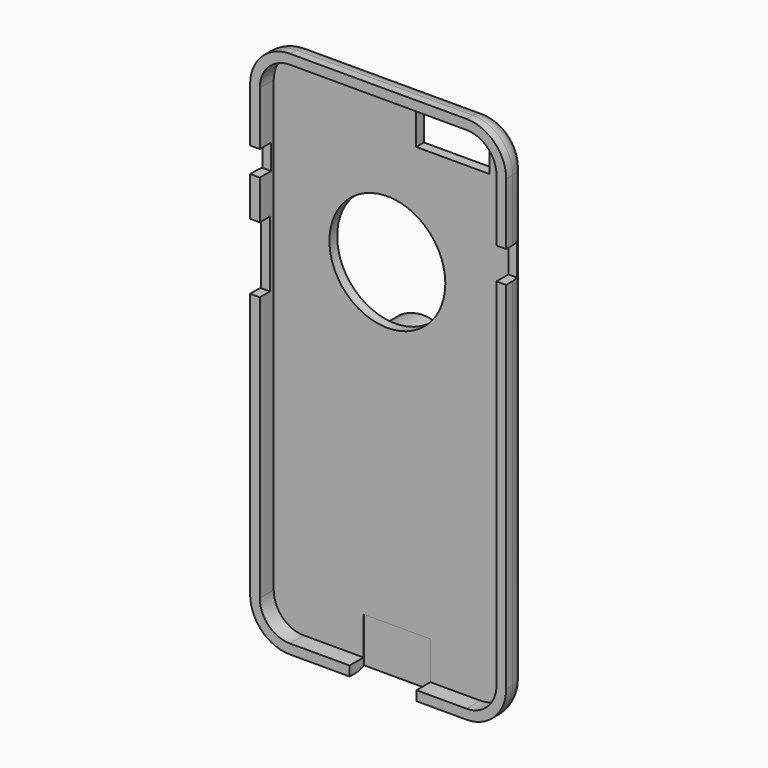
from build123d import *

# Parameters (mm, degrees)
F0_W          = 67.1
F0_H          = 138.6
F1_DEPTH      = 7.1
F2_R          = 10.4245741623
F3_T          = -2.54
F4_W          = 19.2213095725
F4_H          = 9.1803260148
F5_DEPTH      = 12.5
F6_W          = 17.5000010058
F6_H          = 4.661475262
F7_DEPTH      = 12.5
F8_W          = 3.0759498477
F8_H          = 14.1388773918
F9_DEPTH      = 12.5
F10_W         = 3.7169439722
F10_H         = 6.5781623125
F11_DEPTH     = 12.5
F12_W         = 3.3410489097
F12_H         = 17.2911705449
F13_DEPTH     = 12.5
F14_W         = 3.904892784
F14_H         = 8.2696899772
F15_DEPTH     = 12.5
F16_T1_DEPTH  = 117.7508516753
F16_T3_DEPTH  = 46.2508516753
F16_T6_ANGLE  = 90
F16_T8_ANGLE  = 90
F16_T10_ANGLE = 90
F16_T12_ANGLE = 90
F17_R         = 15.1895589548
F18_DEPTH     = 12.5
F19_R         = 10.4830955048
F19_R_2       = 9.0277735867
F20_DEPTH     = 7.7


# Not quite as in the source:
# - a fillet or chamfer that OpenCascade refuses, or shapes differently, is made with other operations: its cross-section is extruded or revolved along the edge and cut away or added


with BuildPart() as f1:
    # F0 (on Front) → F1 (new body)
    with BuildSketch(Plane.XZ):
        Rectangle(F0_W, F0_H)
    extrude(amount=F1_DEPTH)

    # F2
    f2_edges = [f1.edges().sort_by_distance(p)[0] for p in [
        (33.55, -3.55, 69.3),
        (-33.55, -3.55, 69.3),
        (-33.55, -3.55, -69.3),
        (33.55, -3.55, -69.3),
    ]]
    fillet(f2_edges, radius=F2_R)

    # F3
    f3_openings = [f1.faces().sort_by_distance(p)[0] for p in [
        (0, -7.1, 0),
    ]]
    offset(amount=F3_T, openings=f3_openings)

    # F4 (on Front) → F5 (cut, symmetric)
    with BuildSketch(Plane.XZ):
        with Locations((15.9221310169, 60.1024609059)):
            Rectangle(F4_W, F4_H)
    extrude(amount=F5_DEPTH, both=True, mode=Mode.SUBTRACT)

    # F6 (on face) → F7 (cut, symmetric)
    with BuildSketch(Plane(origin=(0, 0, -69.3), x_dir=(1, 0, 0), z_dir=(0, 0, -1))):
        with Locations((1.2909830548, 4.769262369)):
            Rectangle(F6_W, F6_H)
    extrude(amount=F7_DEPTH, both=True, mode=Mode.SUBTRACT)

    # F8 (on Front) → F9 (cut, symmetric)
    with BuildSketch(Plane.XZ):
        with Locations((35.5030968785, 36.7480814457)):
            Rectangle(F8_W, F8_H)
    extrude(amount=F9_DEPTH, both=True, mode=Mode.SUBTRACT)

    # F10 (on face) → F11 (cut, symmetric)
    with BuildSketch(Plane(origin=(-33.55, 0, 0), x_dir=(0, -1, 0), z_dir=(-1, 0, 0))):
        with Locations((5.2415280139, 41.4424240589)):
            Rectangle(F10_W, F10_H)
    extrude(amount=F11_DEPTH, both=True, mode=Mode.SUBTRACT)

    # F12 (on face) → F13 (cut, symmetric)
    with BuildSketch(Plane(origin=(-33.55, 0, 0), x_dir=(0, -1, 0), z_dir=(-1, 0, 0))):
        with Locations((5.4294755451, 19.1706451587)):
            Rectangle(F12_W, F12_H)
    extrude(amount=F13_DEPTH, both=True, mode=Mode.SUBTRACT)

    # F14 (on face) → F15 (cut, symmetric)
    with BuildSketch(Plane.YZ.offset(33.55)):
        with Locations((-5.147553608, 38.5292358696)):
            Rectangle(F14_W, F14_H)
    extrude(amount=F15_DEPTH, both=True, mode=Mode.SUBTRACT)

    # F16: fillet of radius 5 on 1 edges, made by hand

    # F16_s2 → F16_t1 (cut)
    with BuildSketch(Plane.XY.offset(-58.8754258377)):
        with BuildLine():
            ThreePointArc((33.55, -5), (32.0855339059, -1.4644660941), (28.55, 0))
            Line((28.55, 0), (33.55, 0))
            Line((33.55, 0), (33.55, -5))
        make_face()
        with BuildLine():
            ThreePointArc((-28.55, 0), (-32.0855339059, -1.4644660941), (-33.55, -5))
            Line((-33.55, -5), (-33.55, 0))
            Line((-33.55, 0), (-28.55, 0))
        make_face()
    extrude(amount=F16_T1_DEPTH, mode=Mode.SUBTRACT)

    # F16_s4 → F16_t3 (cut)
    with BuildSketch(Plane.YZ.offset(-23.1254258377)):
        with BuildLine():
            ThreePointArc((0, 64.3), (-1.4644660941, 67.8355339059), (-5, 69.3))
            Line((-5, 69.3), (0, 69.3))
            Line((0, 69.3), (0, 64.3))
        make_face()
        with BuildLine():
            ThreePointArc((0, -64.3), (-1.4644660941, -67.8355339059), (-5, -69.3))
            Line((-5, -69.3), (0, -69.3))
            Line((0, -69.3), (0, -64.3))
        make_face()
    extrude(amount=F16_T3_DEPTH, mode=Mode.SUBTRACT)

    # F16_s5 → F16_t6 (revolve, cut)
    with BuildSketch(Plane.XY.offset(-58.8754258377)):
        with BuildLine():
            ThreePointArc((28.55, 0), (32.0855339059, -1.4644660941), (33.55, -5))
            Line((33.55, -5), (33.55, 0))
            Line((33.55, 0), (28.55, 0))
        make_face()
    revolve(axis=Axis((23.1254258377, 0, -58.8754258377), (0, 1, 0)), revolution_arc=F16_T6_ANGLE, mode=Mode.SUBTRACT)

    # F16_s7 → F16_t8 (revolve, cut)
    with BuildSketch(Plane.XY.offset(58.8754258377)):
        with BuildLine():
            ThreePointArc((28.55, 0), (32.0855339059, -1.4644660941), (33.55, -5))
            Line((33.55, -5), (33.55, 0))
            Line((33.55, 0), (28.55, 0))
        make_face()
    revolve(axis=Axis((23.1254258377, 0, 58.8754258377), (0, -1, 0)), revolution_arc=F16_T8_ANGLE, mode=Mode.SUBTRACT)

    # F16_s9 → F16_t10 (revolve, cut)
    with BuildSketch(Plane.YZ.offset(-23.1254258377)):
        with BuildLine():
            ThreePointArc((0, 64.3), (-1.4644660941, 67.8355339059), (-5, 69.3))
            Line((-5, 69.3), (0, 69.3))
            Line((0, 69.3), (0, 64.3))
        make_face()
    revolve(axis=Axis((-23.1254258377, 0, 58.8754258377), (0, -1, 0)), revolution_arc=F16_T10_ANGLE, mode=Mode.SUBTRACT)

    # F16_s11 → F16_t12 (revolve, cut)
    with BuildSketch(Plane.XY.offset(-58.8754258377)):
        with BuildLine():
            ThreePointArc((-28.55, 0), (-32.0855339059, -1.4644660941), (-33.55, -5))
            Line((-33.55, -5), (-33.55, 0))
            Line((-33.55, 0), (-28.55, 0))
        make_face()
    revolve(axis=Axis((-23.1254258377, 0, -58.8754258377), (0, -1, 0)), revolution_arc=F16_T12_ANGLE, mode=Mode.SUBTRACT)

    # F17 (on Front) → F18 (cut, symmetric)
    with BuildSketch(Plane.XZ):
        with Locations((-1.2289978711, 26.4862392154)):
            Circle(F17_R)
    extrude(amount=F18_DEPTH, both=True, mode=Mode.SUBTRACT)

    # F19 (on Front) → F20 (join)
    with BuildSketch(Plane.XZ):
        Circle(F19_R)
        Circle(F19_R_2, mode=Mode.SUBTRACT)
    extrude(amount=-F20_DEPTH)


solid = f1.part
